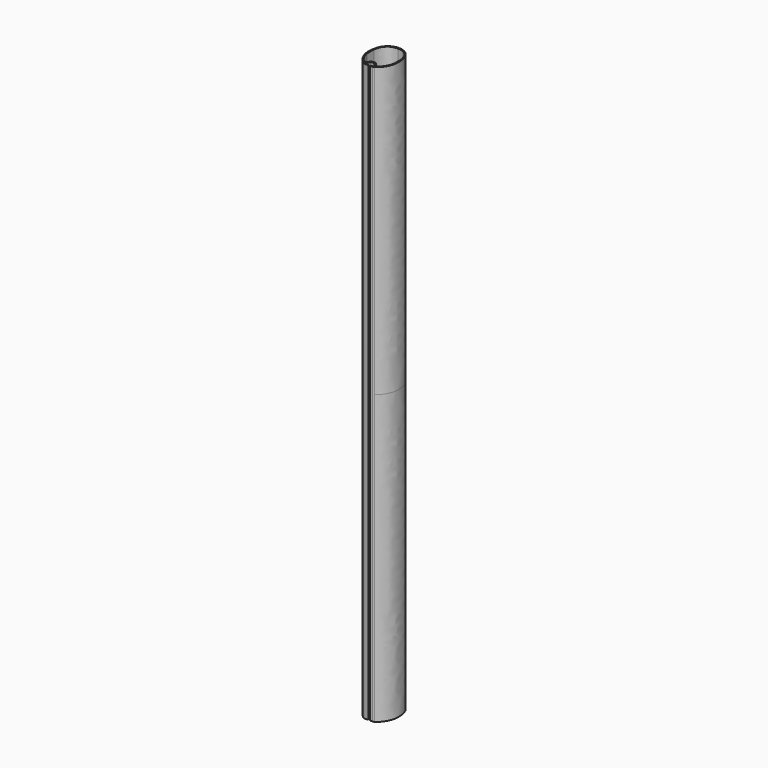
from build123d import *

# Parameters (mm, degrees)
F39_DEPTH = 500


# Not quite as in the source:
# - ends of sketch curves that miss each other by under 0.0002 mm in the source are joined
# - the dataset's text gives a spline's control points without its knots; the knots are read off the source's solid


with BuildPart() as f39:
    # F38 (on Top) → F39 (new body, symmetric)
    with BuildSketch(Plane.XY):
        with BuildLine():
            add(Edge.make_bspline(
                [(23.5536252439, -7.2560820689), (23.5916575277, -7.0510155186), (23.8276840859, -5.7285801466), (24.151531204, -3.4405425007), (24.2873354627, 0.0045356218), (24.1117663849, 3.5050942757), (23.8610925563, 5.9823472927), (23.6100352496, 7.5865837212), (23.5536252439, 7.9230804137)],
                knots=[0.3186426008, 0.3186426008, 0.3186426008, 0.3186426008, 0.3271509051, 0.3740120146, 0.4221074254, 0.470491793, 0.5190548883, 0.5316055523, 0.5316055523, 0.5316055523, 0.5316055523], degree=3))
            Line((23.5536252439, 7.9230804137), (23.5536252439, -7.2560820689))
        make_face()
        with BuildLine():
            add(Edge.make_bspline(
                [(23.5536252439, 7.9230804137), (23.3535723029, 9.1164352465), (22.7597905279, 12.0320516667), (21.3465817892, 16.2721643952), (20.1231279838, 19.6261912332), (16.4356824211, 24.5114069492), (13.7127379229, 26.7043091505), (10.3841309989, 28.7956424718), (9.773572616, 28.9766037477), (8.9376576345, 29.2783622476), (3.7889602927, 30.5452921709), (1.302451708, 30.4786855511), (0, 30.5401328951)],
                knots=[0.5316055523, 0.5316055523, 0.5316055523, 0.5316055523, 0.5761153378, 0.6328393344, 0.682645192, 0.7455304274, 0.7970374007, 0.8467032515, 0.866023277, 0.8889592796, 0.9477441186, 1, 1, 1, 1], degree=3))
            add(Edge.make_bspline(
                [(23.5536252439, -7.2560820689), (23.5916575277, -7.0510155186), (23.8276840859, -5.7285801466), (24.151531204, -3.4405425007), (24.2873354627, 0.0045356218), (24.1117663849, 3.5050942757), (23.8610925563, 5.9823472927), (23.6100352496, 7.5865837212), (23.5536252439, 7.9230804137)],
                knots=[0.3186426008, 0.3186426008, 0.3186426008, 0.3186426008, 0.3271509051, 0.3740120146, 0.4221074254, 0.470491793, 0.5190548883, 0.5316055523, 0.5316055523, 0.5316055523, 0.5316055523], degree=3))
            add(Edge.make_bspline(
                [(10.4187816513, -28.9676227186), (11.7079480537, -27.8705466503), (14.2798804978, -25.524341373), (16.9896606837, -22.1669330847), (19.7261757434, -18.0327940785), (21.4055652093, -14.3241703193), (22.8387426956, -10.682035896), (23.3634012153, -8.2817524061), (23.5536252439, -7.2560820689)],
                knots=[0, 0, 0, 0, 0.058880315, 0.1132859678, 0.1706925161, 0.2233654006, 0.2760870729, 0.3186426008, 0.3186426008, 0.3186426008, 0.3186426008], degree=3))
            Line((10.4187816513, -28.9676227186), (5.5538222126, -23.1697898298))
            ThreePointArc((5.5538222126, -23.1697898298), (3.0639823976, -21.259268544), (0, -20.58))
            Line((0, -20.58), (0, -22.83))
            ThreePointArc((0, -22.83), (2.1130913087, -23.2984610648), (3.8302222156, -24.6160619516))
            Line((3.8302222156, -24.6160619516), (8.4684793359, -30.1437215381))
            add(Edge.make_bspline(
                [(6.65, -31), (6.9546709761, -30.9966091233), (7.5237272259, -30.986551741), (8.2526497082, -30.8785634822), (8.5677592682, -30.5766291439), (8.5882944986, -30.308438465), (8.4684793359, -30.1437215381)],
                knots=[0, 0, 0, 0, 0.3103717511, 0.5865434938, 0.7878644935, 1, 1, 1, 1], degree=3))
            Line((6.65, -31), (3.6160254038, -31))
            ThreePointArc((3.6160254038, -31), (1.8839745962, -31), (2.75, -32.5))
            Line((2.75, -32.5), (6.651236125, -32.5))
            ThreePointArc((6.651236125, -32.5), (8.2194575025, -32.2910968864), (9.6785597859, -31.679558439))
            add(Edge.make_bspline(
                [(9.6785597859, -31.679558439), (9.8583466831, -31.5494218056), (10.3573106888, -31.2000120159), (11.7685158522, -30.1752223914), (15.9045281436, -26.4550937747), (18.5102412317, -23.1048992369), (21.3018526526, -18.8533002992), (23.0908511796, -14.8680295144), (24.5762038864, -10.8243676385), (25.4571270478, -6.9049689645), (25.9275546529, -3.5765491621), (26.0602665892, 0.010692974), (25.8532484214, 3.5904923565), (25.5119778323, 7.2789042864), (24.5952289289, 11.9872035624), (23.0816948011, 16.7893773271), (21.6758529103, 20.3283042369), (17.7857526132, 25.6160368107), (14.5902915982, 28.2986957957), (10.6496706242, 30.6827786965), (7.6444852195, 31.797515139), (3.9605288614, 32.8064243338), (1.3395062246, 32.9497309259), (0, 32.99)],
                knots=[0, 0, 0, 0, 0.0208246159, 0.0522741473, 0.1088331021, 0.1601901023, 0.2139478807, 0.264692263, 0.3147687341, 0.3630227357, 0.40725525, 0.4528163776, 0.4983842129, 0.5447305457, 0.5979548116, 0.6516566578, 0.6994229663, 0.7603409694, 0.8108170161, 0.8616415521, 0.9050756214, 0.9517331874, 1, 1, 1, 1], degree=3))
            Line((0, 32.99), (0, 30.5401328951))
        make_face()
    extrude(amount=F39_DEPTH, both=True)


with BuildPart() as f40_1:
    # F40: instance of F39
    add(f39.part.mirror(Plane.YZ))


with BuildPart() as f39_1:
    add(f39.part)

    # F41: union F40_1
    add(f40_1.part)


solid = f39_1.part
